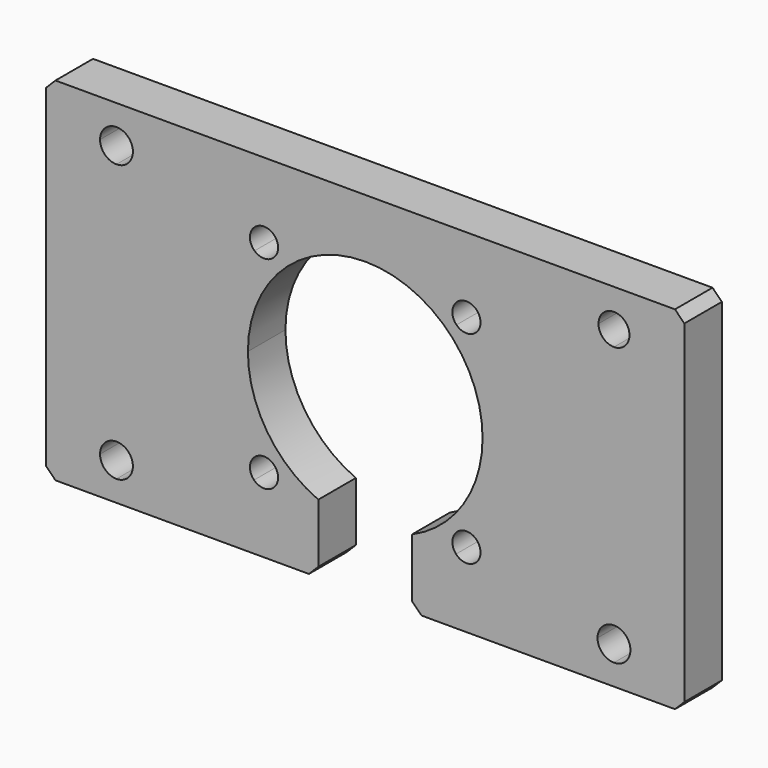
from build123d import *

# Parameters (mm, degrees)
F1_DEPTH = 10


# Not quite as in the source:
# - ends of sketch curves that miss each other by under 0.0002 mm in the source are joined


with BuildPart() as f1:
    # F0 (on Front) → F1 (new body)
    with BuildSketch(Plane.XZ):
        with BuildLine():
            Line((-28.537618, -30.289698), (25.462382, -30.289698))
            Line((25.462382, -30.289698), (27.462382, -28.289698))
            Line((27.462382, -28.289698), (27.462382, 42.710302))
            Line((27.462382, 42.710302), (25.462382, 44.710302))
            Line((25.462382, 44.710302), (-106.537618, 44.710302))
            Line((-106.537618, 44.710302), (-108.537618, 42.710302))
            Line((-108.537618, 42.710302), (-108.537618, -28.289698))
            Line((-108.537618, -28.289698), (-106.537618, -30.289698))
            Line((-106.537618, -30.289698), (-52.537618, -30.289698))
            Line((-52.537618, -30.289698), (-50.537618, -28.289698))
            Line((-50.537618, -28.289698), (-50.537618, -21.6037570684))
            ThreePointArc((-50.537618, -21.6037570684), (-55.4409257201, -19.4006246843), (-59.881294185, -16.3708809994))
            ThreePointArc((-59.881294185, -16.3708809994), (-62.0305817628, -17.3555463136), (-64.2256943436, -16.4777743436))
            ThreePointArc((-64.2256943436, -16.4777743436), (-65.1034663136, -14.2826617628), (-64.1188009994, -12.133374185))
            ThreePointArc((-64.1188009994, -12.133374185), (-69.2558707453, -3.0615994432), (-71.037618, 7.210302))
            ThreePointArc((-71.037618, 7.210302), (-69.2558706203, 17.4822037925), (-64.1188005289, 26.5539787586))
            ThreePointArc((-64.1188005289, 26.5539787586), (-65.1034663058, 28.7032664454), (-64.2256943436, 30.8983793436))
            ThreePointArc((-64.2256943436, 30.8983793436), (-62.0305813759, 31.7761513041), (-59.8812936652, 30.7914854258))
            ThreePointArc((-59.8812936652, 30.7914854258), (-50.8095191267, 35.9285548585), (-40.537618, 37.710302))
            ThreePointArc((-40.537618, 37.710302), (-30.265716524, 35.9285547335), (-21.1939417612, 30.7914849552))
            ThreePointArc((-21.1939417612, 30.7914849552), (-19.0446539415, 31.7761512963), (-16.8495406564, 30.8983793436))
            ThreePointArc((-16.8495406564, 30.8983793436), (-16.1992224025, 29.9251092971), (-15.970861, 28.777059))
            ThreePointArc((-15.970861, 28.777059), (-16.2283003475, 27.5611802778), (-16.9564350448, 26.5539782388))
            ThreePointArc((-16.9564350448, 26.5539782388), (-11.8193652665, 17.482203476), (-10.037618, 7.210302))
            ThreePointArc((-10.037618, 7.210302), (-11.8193651415, -3.0615991267), (-16.9564345742, -12.1333736652))
            ThreePointArc((-16.9564345742, -12.1333736652), (-16.2283002188, -13.140575568), (-15.970861, -14.356454))
            ThreePointArc((-15.970861, -14.356454), (-16.1992224025, -15.5045042971), (-16.8495406564, -16.4777743436))
            ThreePointArc((-16.8495406564, -16.4777743436), (-19.0446535546, -17.3555463058), (-21.1939412414, -16.3708805289))
            ThreePointArc((-21.1939412414, -16.3708805289), (-25.6343099562, -19.4006245031), (-30.537618, -21.6037570684))
            Line((-30.537618, -21.6037570684), (-30.537618, -28.289698))
            Line((-30.537618, -28.289698), (-28.537618, -30.289698))
        make_face()
        with BuildLine():
            ThreePointArc((-93.537618, -18.789698), (-91.0627442658, -19.8148242658), (-90.037618, -22.289698))
            ThreePointArc((-90.037618, -22.289698), (-91.0627442658, -24.7645717342), (-93.537618, -25.789698))
            ThreePointArc((-93.537618, -25.789698), (-96.0124917342, -24.7645717342), (-97.037618, -22.289698))
            ThreePointArc((-97.037618, -22.289698), (-96.0124917342, -19.8148242658), (-93.537618, -18.789698))
        make_face(mode=Mode.SUBTRACT)
        with BuildLine():
            ThreePointArc((12.462382, -18.789698), (14.9372557342, -19.8148242658), (15.962382, -22.289698))
            ThreePointArc((15.962382, -22.289698), (14.9372557342, -24.7645717342), (12.462382, -25.789698))
            ThreePointArc((12.462382, -25.789698), (9.9875082658, -24.7645717342), (8.962382, -22.289698))
            ThreePointArc((8.962382, -22.289698), (9.9875082658, -19.8148242658), (12.462382, -18.789698))
        make_face(mode=Mode.SUBTRACT)
        with BuildLine():
            ThreePointArc((-93.537618, 40.210302), (-91.0627442658, 39.1851757342), (-90.037618, 36.710302))
            ThreePointArc((-90.037618, 36.710302), (-91.0627442658, 34.2354282658), (-93.537618, 33.210302))
            ThreePointArc((-93.537618, 33.210302), (-96.0124917342, 34.2354282658), (-97.037618, 36.710302))
            ThreePointArc((-97.037618, 36.710302), (-96.0124917342, 39.1851757342), (-93.537618, 40.210302))
        make_face(mode=Mode.SUBTRACT)
        with BuildLine():
            ThreePointArc((12.462382, 33.410302), (10.1289296221, 34.3768496221), (9.162382, 36.710302))
            ThreePointArc((9.162382, 36.710302), (10.1289296221, 39.0437543779), (12.462382, 40.010302))
            ThreePointArc((12.462382, 40.010302), (14.7958343779, 39.0437543779), (15.762382, 36.710302))
            ThreePointArc((15.762382, 36.710302), (14.7958343779, 34.3768496221), (12.462382, 33.410302))
        make_face(mode=Mode.SUBTRACT)
        with BuildLine():
            ThreePointArc((-40.537618, 32.210302), (-22.8599484703, 24.8879715297), (-15.537618, 7.210302))
            Line((-15.537618, 7.210302), (-10.037618, 7.210302))
            ThreePointArc((-10.037618, 7.210302), (-11.8193652665, 17.482203476), (-16.9564350448, 26.5539782388))
            ThreePointArc((-16.9564350448, 26.5539782388), (-19.0446539415, 25.7779667037), (-21.0921813436, 26.6557386564))
            ThreePointArc((-21.0921813436, 26.6557386564), (-21.9699532963, 28.7032660585), (-21.1939417612, 30.7914849552))
            ThreePointArc((-21.1939417612, 30.7914849552), (-30.265716524, 35.9285547335), (-40.537618, 37.710302))
            Line((-40.537618, 37.710302), (-40.537618, 32.210302))
        make_face()
        with BuildLine():
            ThreePointArc((-65.537618, 7.210302), (-58.2152875297, 24.8879715297), (-40.537618, 32.210302))
            Line((-40.537618, 32.210302), (-40.537618, 37.710302))
            ThreePointArc((-40.537618, 37.710302), (-50.8095191267, 35.9285548585), (-59.8812936652, 30.7914854258))
            ThreePointArc((-59.8812936652, 30.7914854258), (-59.3053347894, 29.8565864419), (-59.104374, 28.777059))
            ThreePointArc((-59.104374, 28.777059), (-59.3327354025, 27.6290087029), (-59.9830536564, 26.6557386564))
            ThreePointArc((-59.9830536564, 26.6557386564), (-62.0305814454, 25.7779666942), (-64.1188005289, 26.5539787586))
            ThreePointArc((-64.1188005289, 26.5539787586), (-69.2558706203, 17.4822037925), (-71.037618, 7.210302))
            Line((-71.037618, 7.210302), (-65.537618, 7.210302))
        make_face()
        with BuildLine():
            ThreePointArc((-59.881294185, -16.3708809994), (-55.4409257201, -19.4006246843), (-50.537618, -21.6037570684))
            Line((-50.537618, -21.6037570684), (-50.537618, -15.702576))
            ThreePointArc((-50.537618, -15.702576), (-61.4541187154, -6.4827618582), (-65.537618, 7.210302))
            Line((-65.537618, 7.210302), (-71.037618, 7.210302))
            ThreePointArc((-71.037618, 7.210302), (-69.2558707453, -3.0615994432), (-64.1188009994, -12.133374185))
            ThreePointArc((-64.1188009994, -12.133374185), (-62.0305817628, -11.3573616864), (-59.9830536564, -12.2351336564))
            ThreePointArc((-59.9830536564, -12.2351336564), (-59.3327354025, -13.2084037029), (-59.104374, -14.356454))
            ThreePointArc((-59.104374, -14.356454), (-59.3053349287, -15.435981803), (-59.881294185, -16.3708809994))
        make_face()
        with BuildLine():
            Line((-30.537618, -15.702576), (-30.537618, -21.6037570684))
            ThreePointArc((-30.537618, -21.6037570684), (-25.6343099562, -19.4006245031), (-21.1939412414, -16.3708805289))
            ThreePointArc((-21.1939412414, -16.3708805289), (-21.9699533058, -14.2826614454), (-21.0921813436, -12.2351336564))
            ThreePointArc((-21.0921813436, -12.2351336564), (-19.0446536241, -11.3573616959), (-16.9564345742, -12.1333736652))
            ThreePointArc((-16.9564345742, -12.1333736652), (-11.8193651415, -3.0615991267), (-10.037618, 7.210302))
            Line((-10.037618, 7.210302), (-15.537618, 7.210302))
            ThreePointArc((-15.537618, 7.210302), (-19.6211172846, -6.4827618582), (-30.537618, -15.702576))
        make_face()
    extrude(amount=-F1_DEPTH)


solid = f1.part
